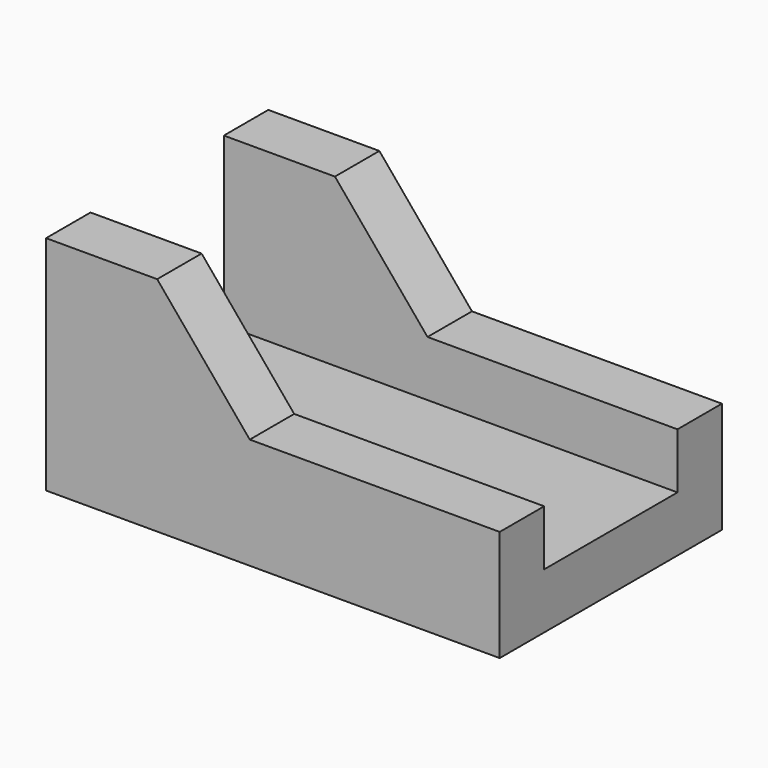
from build123d import *

# Parameters (mm, degrees)
F0_W     = 77.7875
F0_H     = 47.625
F1_DEPTH = 9.525
F3_DEPTH = 9.525


# Not quite as in the source:
# - a pattern or mirror of a feature is missing from the dataset's text; its kind, count and spacing are read off the source's solid


with BuildPart() as f1:
    # F0 (on Top) → F1 (new body)
    with BuildSketch(Plane.XY):
        Rectangle(F0_W, F0_H)
    extrude(amount=F1_DEPTH)

    # F2 (on face) → F3 (join)
    with BuildSketch(Plane.XZ.offset(23.8125)):
        Polygon((-38.89375, 38.1), (-38.89375, 9.525), (38.89375, 9.525), (38.89375, 19.05), (-3.96875, 19.05), (-19.84375, 38.1), align=None)
    f3 = extrude(amount=-F3_DEPTH)

    # F3_copies: F3 across plane
    add(f3.mirror(Plane.ZX))


solid = f1.part
